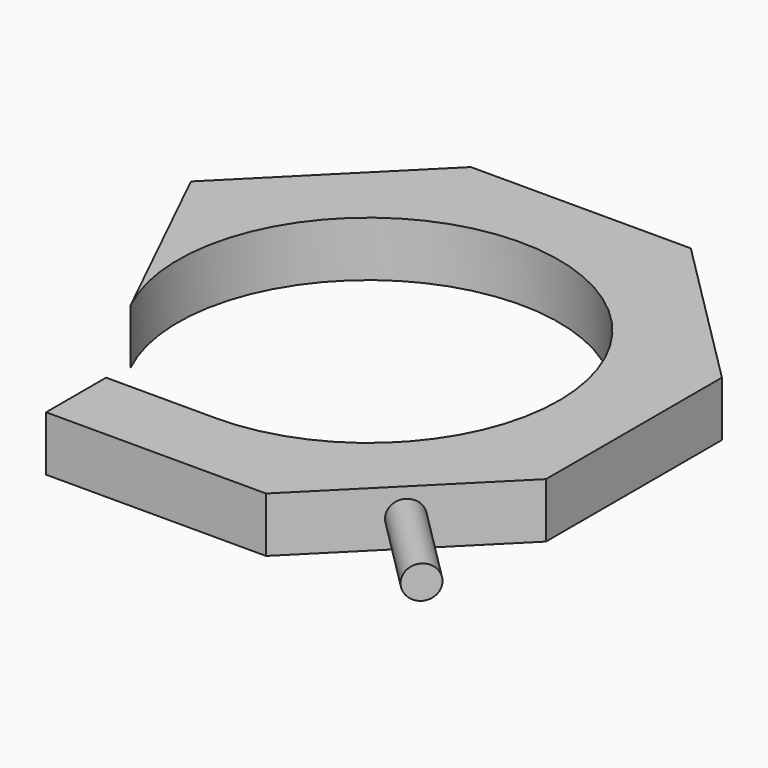
from build123d import *

# Parameters (mm, degrees)
F1_DEPTH = 3.175
F2_R     = 0.9525
F3_DEPTH = 6.35


# Not quite as in the source:
# - a length typed as a fraction of an inch, garbled in the dataset ("3 / 203.2 mm" for 3/8 in), is restored


with BuildPart() as f1:
    # F0 (on Top) → F1 (new body)
    with BuildSketch(Plane.XY):
        with BuildLine():
            Line((0, 4.3302561211), (0, 0))
            Line((0, 0), (12.7, 0))
            Line((12.7, 0), (15.24, 2.54))
            Line((15.24, 2.54), (21.6802561211, 8.9802561211))
            Line((21.6802561211, 8.9802561211), (21.6802561211, 21.6802561211))
            Line((21.6802561211, 21.6802561211), (12.7, 30.6605122421))
            Line((12.7, 30.6605122421), (0, 30.6605122421))
            Line((0, 30.6605122421), (-2.54, 28.1205122421))
            Line((-2.54, 28.1205122421), (-8.9802561211, 21.6802561211))
            Line((-8.9802561211, 21.6802561211), (-3.5386407003, 10.5120837393))
            ThreePointArc((-3.5386407003, 10.5120837393), (12.1809563452, 24.657632392), (6.35, 4.3302561211))
            Line((6.35, 4.3302561211), (0, 4.3302561211))
        make_face()
    extrude(amount=F1_DEPTH)

    # F2 (on face) → F3 (join)
    with BuildSketch(Plane(origin=(6.35, -6.35, 0), x_dir=(0.7071067812, 0.7071067812, 0), z_dir=(0.7071067812, -0.7071067812, 0))):
        with Locations((15.3302561211, 1.5875)):
            Circle(F2_R)
    extrude(amount=F3_DEPTH)


solid = f1.part
